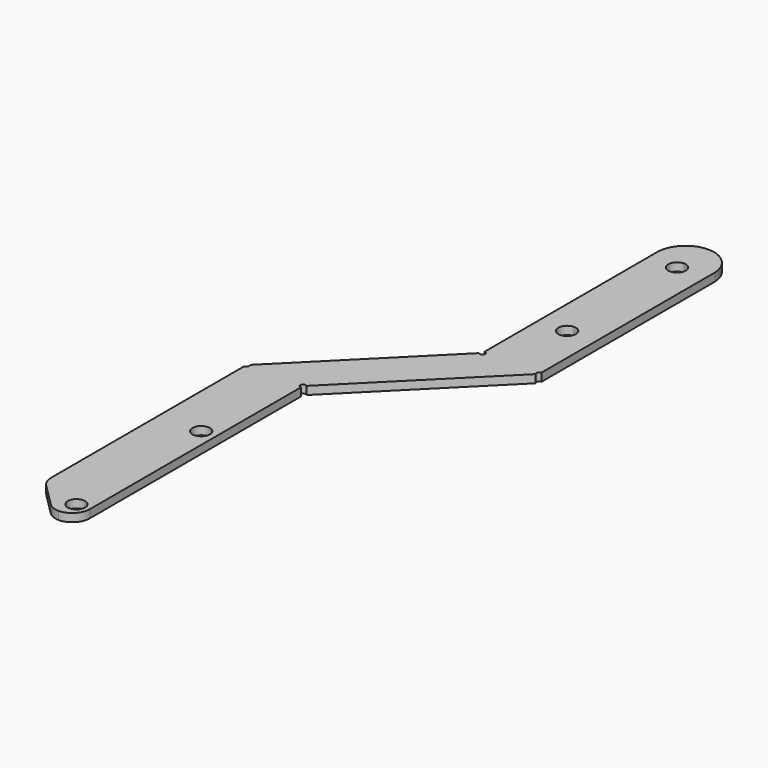
from build123d import *

# Parameters (mm, degrees)
F0_R        = 5.08
F1_DEPTH    = 4.699
F2_T1_DEPTH = 25.7410489686
F2_T3_DEPTH = 55.499


# Not quite as in the source:
# - a fillet or chamfer that OpenCascade refuses, or shapes differently, is made with other operations: its cross-section is extruded or revolved along the edge and cut away or added


with BuildPart() as f1:
    # F0 (on Top) → F1 (new body)
    with BuildSketch(Plane.XY):
        with BuildLine():
            Line((31.4325, 165.1), (1.5875, 165.1))
            ThreePointArc((1.5875, 165.1), (1.1225320151, 163.9774679849), (0, 163.5125))
            Line((0, 163.5125), (0, 19.05))
            Line((0, 19.05), (19.05, 0))
            Line((19.05, 0), (33.02, 0))
            Line((33.02, 0), (33.02, 163.5125))
            ThreePointArc((33.02, 163.5125), (31.8974679849, 163.9774679849), (31.4325, 165.1))
        make_face()
        with Locations((25.2715107054, 10.16)):
            Circle(F0_R, mode=Mode.SUBTRACT)
        with Locations((24.5934482664, 101.6)):
            Circle(F0_R, mode=Mode.SUBTRACT)
        with BuildLine():
            Line((76.2, 368.6610758305), (76.2, 242.8875))
            ThreePointArc((76.2, 242.8875), (77.3225320151, 242.4225320151), (77.7875, 241.3))
            Line((77.7875, 241.3), (92.71, 241.3))
            Line((92.71, 241.3), (92.71, 277.1550263596))
            ThreePointArc((92.71, 277.1550263596), (87.63, 282.2350263596), (92.71, 287.3150263596))
            Line((92.71, 287.3150263596), (92.71, 356.975927515))
            ThreePointArc((92.71, 356.975927515), (87.63, 362.055927515), (92.71, 367.135927515))
            Line((92.71, 367.135927515), (92.71, 384.755953431))
            ThreePointArc((92.71, 384.755953431), (81.1825763095, 380.0653413474), (76.2, 368.6610758305))
        make_face()
        with BuildLine():
            Line((92.71, 277.1550263596), (92.71, 241.3))
            Line((92.71, 241.3), (107.6325, 241.3))
            ThreePointArc((107.6325, 241.3), (108.0974679849, 242.4225320151), (109.22, 242.8875))
            Line((109.22, 242.8875), (109.22, 368.8926994801))
            ThreePointArc((109.22, 368.8926994801), (104.1590146553, 380.148561327), (92.71, 384.755953431))
            Line((92.71, 384.755953431), (92.71, 367.135927515))
            ThreePointArc((92.71, 367.135927515), (96.3021024484, 365.6480299635), (97.79, 362.055927515))
            ThreePointArc((97.79, 362.055927515), (96.3021024484, 358.4638250666), (92.71, 356.975927515))
            Line((92.71, 356.975927515), (92.71, 287.3150263596))
            ThreePointArc((92.71, 287.3150263596), (96.3021024484, 285.827128808), (97.79, 282.2350263596))
            ThreePointArc((97.79, 282.2350263596), (96.3021024484, 278.6429239111), (92.71, 277.1550263596))
        make_face()
        with BuildLine():
            ThreePointArc((1.1225320151, 166.2225320151), (1.4666587579, 165.7075099489), (1.5875, 165.1))
            Line((1.5875, 165.1), (31.4325, 165.1))
            ThreePointArc((31.4325, 165.1), (32.4124900511, 166.5666587579), (34.1425320151, 166.2225320151))
            Line((34.1425320151, 166.2225320151), (108.0974679849, 240.1774679849))
            ThreePointArc((108.0974679849, 240.1774679849), (107.7533412421, 240.6924900511), (107.6325, 241.3))
            Line((107.6325, 241.3), (92.71, 241.3))
            Line((92.71, 241.3), (77.7875, 241.3))
            ThreePointArc((77.7875, 241.3), (76.8075099489, 239.8333412421), (75.0774679849, 240.1774679849))
            Line((75.0774679849, 240.1774679849), (1.1225320151, 166.2225320151))
        make_face()
    extrude(amount=F1_DEPTH)

    # F2: fillet of radius 10.16 on 3 edges, made by hand

    # F2_s2 → F2_t1 (cut)
    with BuildSketch(Plane.XY.offset(-10.5210244843)):
        with BuildLine():
            ThreePointArc((0, 23.2584097937), (0.7733839497, 19.3703461209), (2.9757951031, 16.0742048969))
            Line((2.9757951031, 16.0742048969), (0, 19.05))
            Line((0, 19.05), (0, 23.2584097937))
        make_face()
        with BuildLine():
            ThreePointArc((16.0742048969, 2.9757951031), (19.3703461209, 0.7733839497), (23.2584097937, 0))
            Line((23.2584097937, 0), (19.05, 0))
            Line((19.05, 0), (16.0742048969, 2.9757951031))
        make_face()
    extrude(amount=F2_T1_DEPTH, mode=Mode.SUBTRACT)

    # F2_s4 → F2_t3 (cut)
    with BuildSketch(Plane.XY.offset(-25.4)):
        with BuildLine():
            ThreePointArc((22.86, 0), (30.0442048969, 2.9757951031), (33.02, 10.16))
            Line((33.02, 10.16), (33.02, 0))
            Line((33.02, 0), (22.86, 0))
        make_face()
    extrude(amount=F2_T3_DEPTH, mode=Mode.SUBTRACT)


solid = f1.part
